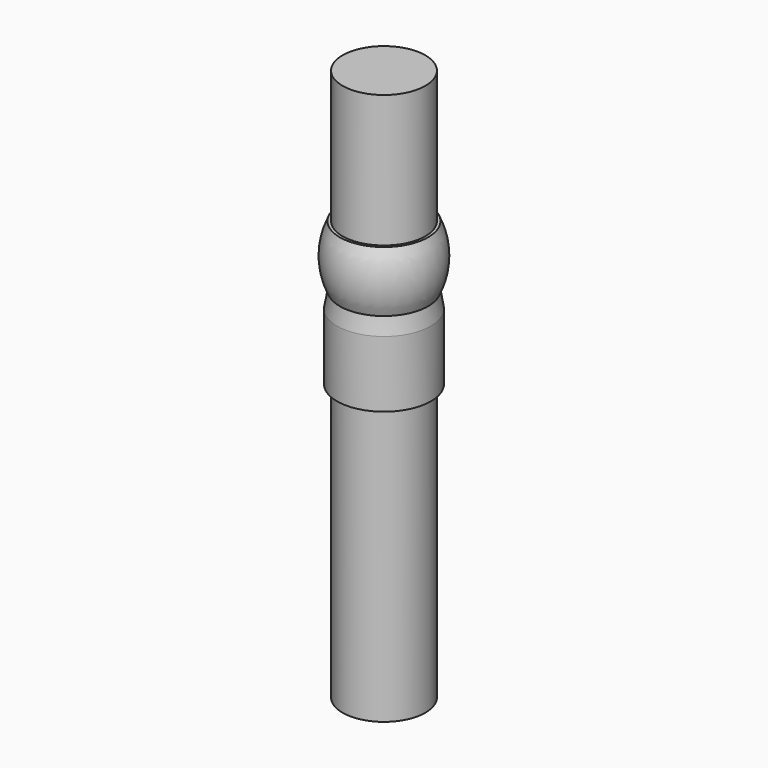
from build123d import *

# Parameters (mm, degrees)
F0_R          = 7.5
F1_DEPTH      = 50
F1_DEPTH_BACK = 50
F2_R          = 8.5
F2_R_2        = 7.5
F3_DEPTH      = 12


with BuildPart() as f1:
    # F0 (on Top) → F1 (new body, two sides)
    with BuildSketch(Plane.XY) as f1_sk:
        Circle(F0_R)
    extrude(amount=F1_DEPTH)
    extrude(f1_sk.sketch, amount=-F1_DEPTH_BACK)


with BuildPart() as f3:
    # F2 (on Top) → F3 (new body)
    with BuildSketch(Plane.XY):
        Circle(F2_R)
        Circle(F2_R_2, mode=Mode.SUBTRACT)
    extrude(amount=F3_DEPTH)

    # F4 (on Front) → F5 (revolve)
    with BuildSketch(Plane.XZ):
        with BuildLine():
            Line((-8, 15), (-7.5, 15))
            Line((-7.5, 15), (-7.5, 22))
            Line((-7.5, 22), (-6.75, 22))
            Line((-6.75, 22), (-6.75, 26))
            Line((-6.75, 26), (-7.5, 26))
            Line((-7.5, 26), (-8, 26))
            ThreePointArc((-8, 26), (-9.25, 20.5), (-8, 15))
        make_face()
        Polygon((-7.5, 12), (-7.5, 15), (-8, 15), (-8.5, 12), align=None)
    revolve(axis=Axis((0, 0, 32.3733808473), (0, 0, -1)))


solid = Compound([f1.part, f3.part])
